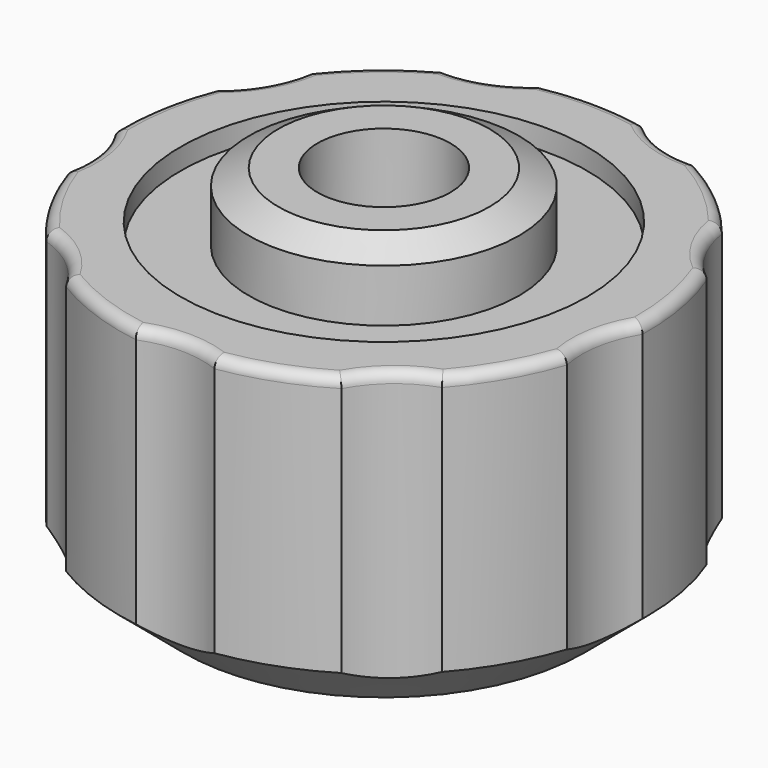
from build123d import *

# Parameters (mm, degrees)
F2_R         = 10
F3_DEPTH     = 30.001
F4_R         = 1
F5_T3_ANGLE  = 72.4183645551
F5_T6_ANGLE  = 34.3109861798
F5_T9_ANGLE  = 34.3109861798
F5_T12_ANGLE = 72.4183645551
F5_T15_ANGLE = 34.3109861798
F5_T18_ANGLE = 72.4183645551
F5_T21_ANGLE = 34.3109861799
F5_T24_ANGLE = 72.4183645551
F5_T27_ANGLE = 34.3109861798
F5_T30_ANGLE = 72.4183645551
F5_T33_ANGLE = 34.3109861799
F5_T36_ANGLE = 72.4183645551
F5_T39_ANGLE = 34.3109861799
F5_T42_ANGLE = 72.4183645551
F5_T45_ANGLE = 34.3109861799
F5_T48_ANGLE = 72.4183645551
F5_T51_ANGLE = 34.3109861798
F5_T54_ANGLE = 72.4183645551


# Not quite as in the source:
# - a fillet or chamfer that OpenCascade refuses, or shapes differently, is made with other operations: its cross-section is extruded or revolved along the edge and cut away or added


with BuildPart() as f1:
    # F0 (on Front) → F1 (revolve)
    with BuildSketch(Plane.XZ):
        Polygon((8, 8), (8.6999093082, 0), (18.6999093082, 0), (25, 5.2864037759), (25, 30), (19.25, 30), (19.25, 28), (12.8, 28), (12.8, 33), (10, 34.5), (6.3, 34.5), (6.3, 24.5), (3.2, 24.5), (3.2, 8), align=None)
    revolve(axis=Axis((0, 0, 15.2192509614), (0, 0, 1)))

    # F2 (on face) → F3 (cut, through all)
    with BuildSketch(Plane.XY.offset(30)):
        with Locations((11.6286848731, 31.9495491067)):
            Circle(F2_R)
        with Locations((-11.6286848731, 31.9495491067)):
            Circle(F2_R)
        with Locations((-29.4448637287, 17)):
            Circle(F2_R)
        with Locations((-33.4834636024, -5.9040380407)):
            Circle(F2_R)
        with Locations((-21.8547787293, -26.045511066)):
            Circle(F2_R)
        with Locations((0, -34)):
            Circle(F2_R)
        with Locations((21.8547787293, -26.045511066)):
            Circle(F2_R)
        with Locations((33.4834636024, -5.9040380407)):
            Circle(F2_R)
        with Locations((29.4448637287, 17)):
            Circle(F2_R)
    extrude(amount=-F3_DEPTH, mode=Mode.SUBTRACT)

    # F4
    f4_edges = [f1.edges().sort_by_distance(p)[0] for p in [
        (-8.699909, 0, 0),
        (-18.699909, 0, 0),
    ]]
    fillet(f4_edges, radius=F4_R)

    # F5: fillet of radius 1 on 18 edges, made by hand


with BuildPart() as f5_tool1:
    # F5_s2 → F5_t3 (revolve)
    with BuildSketch(Plane(origin=(4.7878159953, -19.5059893322, 0), x_dir=(0, 0, 1), z_dir=(0.2383778196, -0.971172495, 0))):
        with BuildLine():
            ThreePointArc((29, 17.4334321252), (29.7071067812, 17.1405389064), (30, 16.4334321252))
            Line((30, 16.4334321252), (30, 17.4334321252))
            Line((30, 17.4334321252), (29, 17.4334321252))
        make_face()
    revolve(axis=Axis((-21.8547787293, -26.045511066, 30), (0, 0, 1)), revolution_arc=F5_T3_ANGLE)


with BuildPart() as f5_tool4:
    # F5_s5 → F5_t6 (revolve)
    with BuildSketch(Plane(origin=(0, 0, 0), x_dir=(0, 0, 1), z_dir=(-0.7969993255, 0.6039801944, 0))):
        with BuildLine():
            ThreePointArc((29, -25), (29.7071067812, -24.7071067812), (30, -24))
            Line((30, -24), (30, -25))
            Line((30, -25), (29, -25))
        make_face()
    revolve(axis=Axis((0, 0, 30), (0, 0, 1)), revolution_arc=F5_T6_ANGLE)


with BuildPart() as f5_tool7:
    # F5_s8 → F5_t9 (revolve)
    with BuildSketch(Plane(origin=(0, 0, 0), x_dir=(0, 0, 1), z_dir=(-0.222305919, 0.974976963, 0))):
        with BuildLine():
            ThreePointArc((29, -25), (29.7071067812, -24.7071067812), (30, -24))
            Line((30, -24), (30, -25))
            Line((30, -25), (29, -25))
        make_face()
    revolve(axis=Axis((0, 0, 30), (0, 0, 1)), revolution_arc=F5_T9_ANGLE)


with BuildPart() as f5_tool10:
    # F5_s11 → F5_t12 (revolve)
    with BuildSketch(Plane(origin=(-8.8705284196, -18.0200035347, 0), x_dir=(0, 0, 1), z_dir=(-0.4416496426, -0.897187602, 0))):
        with BuildLine():
            ThreePointArc((29, 17.4334321252), (29.7071067812, 17.1405389064), (30, 16.4334321252))
            Line((30, 16.4334321252), (30, 17.4334321252))
            Line((30, 17.4334321252), (29, 17.4334321252))
        make_face()
    revolve(axis=Axis((-33.4834636024, -5.9040380407, 30), (0, 0, 1)), revolution_arc=F5_T12_ANGLE)


with BuildPart() as f5_tool13:
    # F5_s14 → F5_t15 (revolve)
    with BuildSketch(Plane(origin=(0, 0, 0), x_dir=(0, 0, 1), z_dir=(0.4564068976, 0.889771175, 0))):
        with BuildLine():
            ThreePointArc((29, -25), (29.7071067812, -24.7071067812), (30, -24))
            Line((30, -24), (30, -25))
            Line((30, -25), (29, -25))
        make_face()
    revolve(axis=Axis((0, 0, 30), (0, 0, 1)), revolution_arc=F5_T15_ANGLE)


with BuildPart() as f5_tool16:
    # F5_s17 → F5_t18 (revolve)
    with BuildSketch(Plane(origin=(-18.378254002, -8.1022578133, 0), x_dir=(0, 0, 1), z_dir=(-0.9150243287, -0.4033986588, 0))):
        with BuildLine():
            ThreePointArc((29, 17.4334321252), (29.7071067812, 17.1405389064), (30, 16.4334321252))
            Line((30, 16.4334321252), (30, 17.4334321252))
            Line((30, 17.4334321252), (29, 17.4334321252))
        make_face()
    revolve(axis=Axis((-29.4448637287, 17, 30), (0, 0, 1)), revolution_arc=F5_T18_ANGLE)


with BuildPart() as f5_tool19:
    # F5_s20 → F5_t21 (revolve)
    with BuildSketch(Plane(origin=(0, 0, 0), x_dir=(0, 0, 1), z_dir=(0.9215618544, 0.3882315655, 0))):
        with BuildLine():
            ThreePointArc((29, -25), (29.7071067812, -24.7071067812), (30, -24))
            Line((30, -24), (30, -25))
            Line((30, -25), (29, -25))
        make_face()
    revolve(axis=Axis((0, 0, 30), (0, 0, 1)), revolution_arc=F5_T21_ANGLE)


with BuildPart() as f5_tool22:
    # F5_s23 → F5_t24 (revolve)
    with BuildSketch(Plane(origin=(-19.2865902853, 5.6066243856, 0), x_dir=(0, 0, 1), z_dir=(-0.960248962, 0.2791450001, 0))):
        with BuildLine():
            ThreePointArc((29, 17.4334321252), (29.7071067812, 17.1405389064), (30, 16.4334321252))
            Line((30, 16.4334321252), (30, 17.4334321252))
            Line((30, 17.4334321252), (29, 17.4334321252))
        make_face()
    revolve(axis=Axis((-11.6286848731, 31.9495491067, 30), (0, 0, 1)), revolution_arc=F5_T24_ANGLE)


with BuildPart() as f5_tool25:
    # F5_s26 → F5_t27 (revolve)
    with BuildSketch(Plane(origin=(0, 0, 0), x_dir=(0, 0, 1), z_dir=(0.9555077776, -0.2949659082, 0))):
        with BuildLine():
            ThreePointArc((29, -25), (29.7071067812, -24.7071067812), (30, -24))
            Line((30, -24), (30, -25))
            Line((30, -25), (29, -25))
        make_face()
    revolve(axis=Axis((0, 0, 30), (0, 0, 1)), revolution_arc=F5_T27_ANGLE)


with BuildPart() as f5_tool28:
    # F5_s29 → F5_t30 (revolve)
    with BuildSketch(Plane(origin=(-11.1705166275, 16.6921047237, 0), x_dir=(0, 0, 1), z_dir=(-0.556162434, 0.8310736111, 0))):
        with BuildLine():
            ThreePointArc((29, 17.4334321252), (29.7071067812, 17.1405389064), (30, 16.4334321252))
            Line((30, 16.4334321252), (30, 17.4334321252))
            Line((30, 17.4334321252), (29, 17.4334321252))
        make_face()
    revolve(axis=Axis((11.6286848731, 31.9495491067, 30), (0, 0, 1)), revolution_arc=F5_T30_ANGLE)


with BuildPart() as f5_tool31:
    # F5_s32 → F5_t33 (revolve)
    with BuildSketch(Plane(origin=(0, 0, 0), x_dir=(0, 0, 1), z_dir=(0.5423609923, -0.8401455553, 0))):
        with BuildLine():
            ThreePointArc((29, -25), (29.7071067812, -24.7071067812), (30, -24))
            Line((30, -24), (30, -25))
            Line((30, -25), (29, -25))
        make_face()
    revolve(axis=Axis((0, 0, 30), (0, 0, 1)), revolution_arc=F5_T33_ANGLE)


with BuildPart() as f5_tool34:
    # F5_s35 → F5_t36 (revolve)
    with BuildSketch(Plane(origin=(2.1723659067, 19.9671637495, 0), x_dir=(0, 0, 1), z_dir=(0.1081586779, 0.9941336431, 0))):
        with BuildLine():
            ThreePointArc((29, 17.4334321252), (29.7071067812, 17.1405389064), (30, 16.4334321252))
            Line((30, 16.4334321252), (30, 17.4334321252))
            Line((30, 17.4334321252), (29, 17.4334321252))
        make_face()
    revolve(axis=Axis((29.4448637287, 17, 30), (0, 0, 1)), revolution_arc=F5_T36_ANGLE)


with BuildPart() as f5_tool37:
    # F5_s38 → F5_t39 (revolve)
    with BuildSketch(Plane(origin=(0, 0, 0), x_dir=(0, 0, 1), z_dir=(-0.4564068976, 0.889771175, 0))):
        with BuildLine():
            ThreePointArc((29, 25), (29.7071067812, 24.7071067812), (30, 24))
            Line((30, 24), (30, 25))
            Line((30, 25), (29, 25))
        make_face()
    revolve(axis=Axis((0, 0, 30), (0, 0, -1)), revolution_arc=F5_T39_ANGLE)


with BuildPart() as f5_tool40:
    # F5_s41 → F5_t42 (revolve)
    with BuildSketch(Plane(origin=(14.49877429, 13.8993649467, 0), x_dir=(0, 0, 1), z_dir=(0.7218711424, 0.692027495, 0))):
        with BuildLine():
            ThreePointArc((29, 17.4334321252), (29.7071067812, 17.1405389064), (30, 16.4334321252))
            Line((30, 16.4334321252), (30, 17.4334321252))
            Line((30, 17.4334321252), (29, 17.4334321252))
        make_face()
    revolve(axis=Axis((33.4834636024, -5.9040380407, 30), (0, 0, 1)), revolution_arc=F5_T42_ANGLE)


with BuildPart() as f5_tool43:
    # F5_s44 → F5_t45 (revolve)
    with BuildSketch(Plane(origin=(0, 0, 0), x_dir=(0, 0, 1), z_dir=(-0.7332018585, -0.6800110548, 0))):
        with BuildLine():
            ThreePointArc((29, -25), (29.7071067812, -24.7071067812), (30, -24))
            Line((30, -24), (30, -25))
            Line((30, -25), (29, -25))
        make_face()
    revolve(axis=Axis((0, 0, 30), (0, 0, 1)), revolution_arc=F5_T45_ANGLE)


with BuildPart() as f5_tool46:
    # F5_s47 → F5_t48 (revolve)
    with BuildSketch(Plane(origin=(20.0410450471, 1.327898811, 0), x_dir=(0, 0, 1), z_dir=(0.9978120766, 0.0661139909, 0))):
        with BuildLine():
            ThreePointArc((29, 17.4334321252), (29.7071067812, 17.1405389064), (30, 16.4334321252))
            Line((30, 16.4334321252), (30, 17.4334321252))
            Line((30, 17.4334321252), (29, 17.4334321252))
        make_face()
    revolve(axis=Axis((21.8547787293, -26.045511066, 30), (0, 0, 1)), revolution_arc=F5_T48_ANGLE)


with BuildPart() as f5_tool49:
    # F5_s50 → F5_t51 (revolve)
    with BuildSketch(Plane(origin=(0, 0, 0), x_dir=(0, 0, 1), z_dir=(-0.9987678899, -0.0496256197, 0))):
        with BuildLine():
            ThreePointArc((29, -25), (29.7071067812, -24.7071067812), (30, -24))
            Line((30, -24), (30, -25))
            Line((30, -25), (29, -25))
        make_face()
    revolve(axis=Axis((0, 0, 30), (0, 0, 1)), revolution_arc=F5_T51_ANGLE)


with BuildPart() as f5_tool52:
    # F5_s53 → F5_t54 (revolve)
    with BuildSketch(Plane(origin=(16.2058880953, -11.8649059363, 0), x_dir=(0, 0, 1), z_dir=(0.8068656507, -0.5907349843, 0))):
        with BuildLine():
            ThreePointArc((29, 17.4334321252), (29.7071067812, 17.1405389064), (30, 16.4334321252))
            Line((30, 16.4334321252), (30, 17.4334321252))
            Line((30, 17.4334321252), (29, 17.4334321252))
        make_face()
    revolve(axis=Axis((0, -34, 30), (0, 0, 1)), revolution_arc=F5_T54_ANGLE)


with BuildPart() as f1_1:
    add(f1.part)

    # F5_t55: cut F5_tool1, F5_tool4, F5_tool7, F5_tool10, F5_tool13, F5_tool16, F5_tool19, F5_tool22, F5_tool25, F5_tool28, F5_tool31, F5_tool34, F5_tool37, F5_tool40, F5_tool43, F5_tool46, F5_tool49, F5_tool52
    add([f5_tool1.part, f5_tool4.part, f5_tool7.part, f5_tool10.part, f5_tool13.part, f5_tool16.part, f5_tool19.part, f5_tool22.part, f5_tool25.part, f5_tool28.part, f5_tool31.part, f5_tool34.part, f5_tool37.part, f5_tool40.part, f5_tool43.part, f5_tool46.part, f5_tool49.part, f5_tool52.part], mode=Mode.SUBTRACT)


solid = f1_1.part
